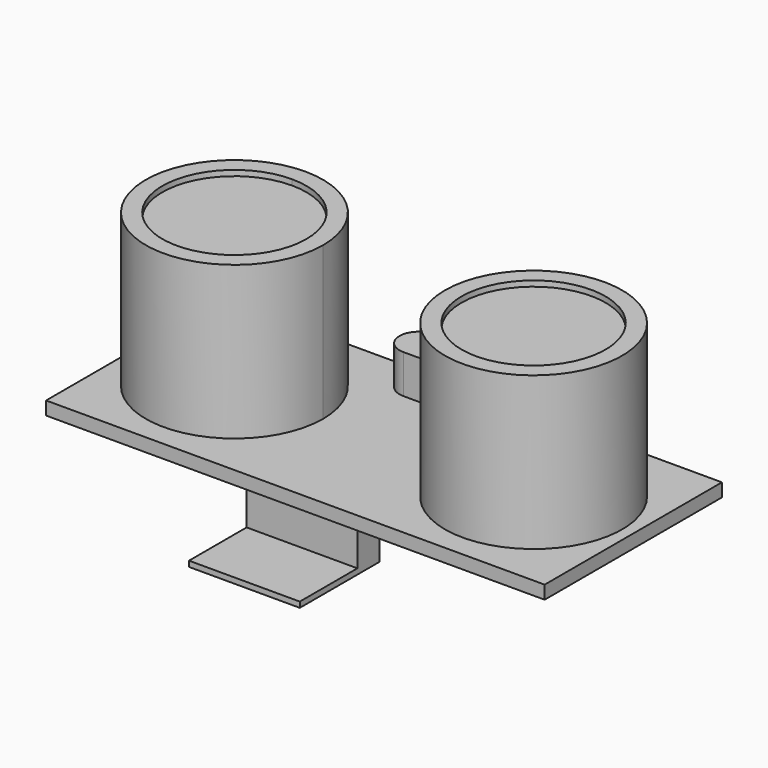
from build123d import *

# Parameters (mm, degrees)
F1_DEPTH = 1.2
F3_DEPTH = 4
F5_DEPTH = 6.5
F7_DEPTH = 13.8
F8_DEPTH = 13.3
F9_DEPTH = 3.5
F10_R    = 1.74999


# Not quite as in the source:
# - a fillet or chamfer is up to 0.001 mm smaller than in the source, because OpenCascade refuses the exact size


with BuildPart() as f1:
    # F0 (on Top) → F1 (new body)
    with BuildSketch(Plane.XY):
        Polygon((9, 0), (0, 0), (0, -20), (45, -20), (45, 0), (36, 0), (22.5, 0), align=None)
    extrude(amount=F1_DEPTH)

    # F2 (on face) → F3 (join)
    with BuildSketch(Plane(origin=(0, 0, 0), x_dir=(1, 0, 0), z_dir=(0, 0, -1))):
        Polygon((22.5, 16.75), (27.5, 16.75), (27.5, 19.25), (17.5, 19.25), (17.5, 16.75), align=None)
    extrude(amount=F3_DEPTH)

    # F4 (on face) → F5 (join)
    with BuildSketch(Plane.XZ.offset(19.25)):
        Polygon((22.5, -3.5), (17.5, -3.5), (17.5, -4), (27.5, -4), (27.5, -3.5), align=None)
    extrude(amount=F5_DEPTH)

    # F6 (on face) → F7 (join)
    with BuildSketch(Plane.XY.offset(1.2)):
        with BuildLine():
            ThreePointArc((44, -10), (36, -2), (28, -10))
            ThreePointArc((28, -10), (36, -18), (44, -10))
        make_face()
        with BuildLine():
            ThreePointArc((42.5, -10), (36, -16.5), (29.5, -10))
            ThreePointArc((29.5, -10), (36, -3.5), (42.5, -10))
        make_face(mode=Mode.SUBTRACT)
        with BuildLine():
            ThreePointArc((17, -10), (14.6568542495, -4.3431457505), (9, -2))
            Line((9, -2), (9, -3.5))
            ThreePointArc((9, -3.5), (13.5961940777, -5.4038059223), (15.5, -10))
            Line((15.5, -10), (17, -10))
        make_face()
        with BuildLine():
            Line((9, -3.5), (9, -2))
            ThreePointArc((9, -2), (3.3431457505, -15.6568542495), (17, -10))
            Line((17, -10), (15.5, -10))
            ThreePointArc((15.5, -10), (4.4038059223, -14.5961940777), (9, -3.5))
        make_face()
    extrude(amount=F7_DEPTH)

    # F8 (add): faces of the model
    f8_faces = [f1.faces().sort_by_distance(p)[0] for p in [
        (9, -10, 1.2),
        (36, -10, 1.2),
    ]]
    extrude(f8_faces, amount=F8_DEPTH)

    # F6 (on face) → F9 (join)
    with BuildSketch(Plane.XY.offset(1.2)):
        Polygon((27.5, -0.25), (22.5, -0.25), (17.5, -0.25), (17.5, -3.75), (27.5, -3.75), align=None)
    extrude(amount=F9_DEPTH)

    # F10 (radius 1.75 in the source; OpenCascade refuses exactly that, so slightly less here)
    f10_edges = [f1.edges().sort_by_distance(p)[0] for p in [
        (27.5, -0.25, 2.95),
        (27.5, -3.75, 2.95),
        (17.5, -0.25, 2.95),
        (17.5, -3.75, 2.95),
    ]]
    fillet(f10_edges, radius=F10_R)


solid = f1.part
